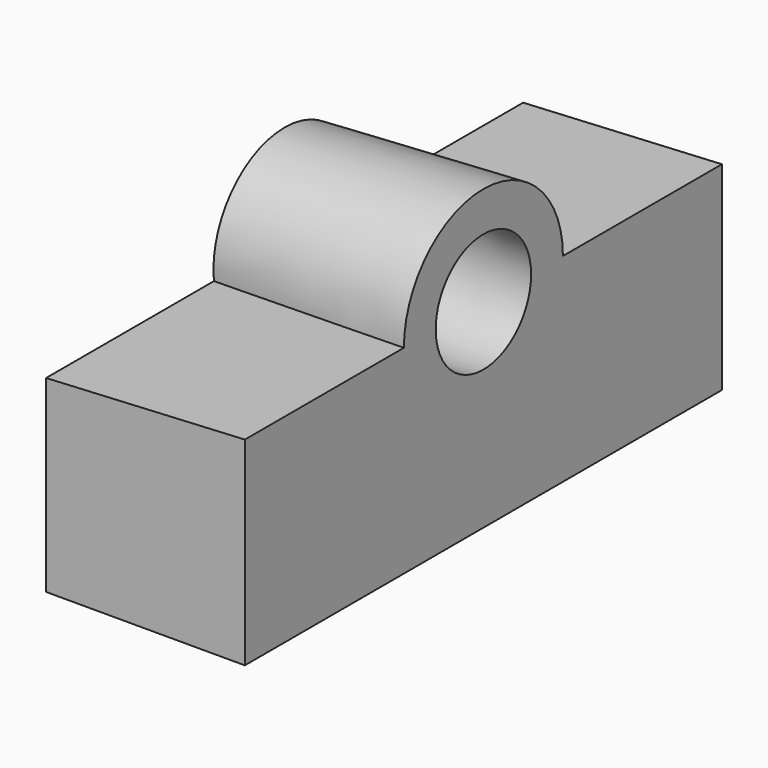
from build123d import *

# Parameters (mm, degrees)
F0_W                   = 76.2
F0_H                   = 50.8
F1_DEPTH               = 25.4
F3_DEPTH               = 25.4
DRAFT_F3_DRAFTED_ANGLE = -3
F4_R                   = 7.62
F5_DEPTH               = 12.7
F5_TAPER               = -3


# Not quite as in the source:
# - an extrude with a draft is written as a straight extrude whose walls are then drafted


with BuildPart() as f1:
    # F0 (on Right) → F1 (new body)
    with BuildSketch(Plane.YZ):
        with Locations((-38.1, 42.5450003982)):
            Rectangle(F0_W, F0_H)
    extrude(amount=F1_DEPTH)


with BuildPart() as f3_drafted:
    # F2 (on face) → F3 (new body)
    with BuildSketch(Plane.YZ.offset(25.4)):
        with BuildLine():
            ThreePointArc((-50.8, 42.5450003982), (-38.1, 55.2450003982), (-25.4, 42.5450003982))
            Line((-25.4, 42.5450003982), (0, 42.5450003982))
            Line((0, 42.5450003982), (0, 67.9450003982))
            Line((0, 67.9450003982), (-76.2, 67.9450003982))
            Line((-76.2, 67.9450003982), (-76.2, 42.5450003982))
            Line((-76.2, 42.5450003982), (-50.8, 42.5450003982))
        make_face()
    extrude(amount=-F3_DEPTH)

    # draft_F3_drafted
    draft_f3_drafted_walls = [f3_drafted.faces().sort_by_distance(p)[0] for p in [
        (8.4666666667, -38.1, 55.2450003982),
        (8.4666666667, -12.7, 42.5450003982),
        (8.4666666667, 0, 55.2450003982),
        (8.4666666667, -38.1, 67.9450003982),
        (8.4666666667, -76.2, 55.2450003982),
        (8.4666666667, -63.5, 42.5450003982),
    ]]
    draft(draft_f3_drafted_walls, neutral_plane=Plane(origin=(25.4, 0, 0), x_dir=(0, 1, 0), z_dir=(-1, 0, 0)), angle=DRAFT_F3_DRAFTED_ANGLE)


with BuildPart() as f1_1:
    add(f1.part)

    # join_F3_drafted: cut F3_drafted
    add(f3_drafted.part, mode=Mode.SUBTRACT)

    # F4 (on face) → F5 (cut)
    with BuildSketch(Plane.YZ.offset(25.4)):
        with Locations((-38.1, 42.5450003982)):
            Circle(F4_R)
    extrude(amount=-F5_DEPTH, taper=F5_TAPER, mode=Mode.SUBTRACT)


solid = f1_1.part
